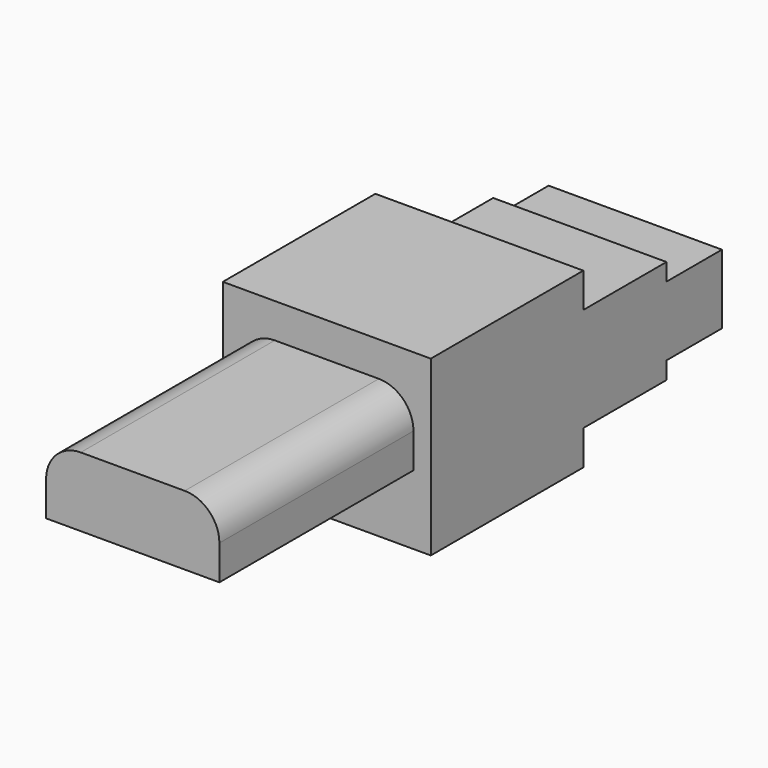
from build123d import *

# Parameters (mm, degrees)
F1_DEPTH = 7
F2_W     = 6
F2_H     = 5
F3_DEPTH = 5.5
F4_W     = 6
F4_H     = 3
F5_DEPTH = 3
F6_W     = 6
F6_H     = 2
F7_DEPTH = 2
F9_DEPTH = 1
F10_SIZE = 0.99999


# Not quite as in the source:
# - a fillet or chamfer is up to 0.001 mm smaller than in the source, because OpenCascade refuses the exact size


with BuildPart() as f1:
    # F0 (on Front) → F1 (new body)
    with BuildSketch(Plane.XZ):
        with BuildLine():
            Line((-2.5, -1), (2.5, -1))
            Line((2.5, -1), (2.5, 0))
            ThreePointArc((2.5, 0), (2.2071067812, 0.7071067812), (1.5, 1))
            Line((1.5, 1), (-1.5, 1))
            ThreePointArc((-1.5, 1), (-2.2071067812, 0.7071067812), (-2.5, 0))
            Line((-2.5, 0), (-2.5, -1))
        make_face()
    extrude(amount=F1_DEPTH)

    # F2 (on face) → F3 (join)
    with BuildSketch(Plane(origin=(0, 0, 0), x_dir=(-1, 0, 0), z_dir=(0, 1, 0))):
        with Locations((0, -0.5)):
            Rectangle(F2_W, F2_H)
        with BuildLine():
            ThreePointArc((1.5, 1), (2.2071067812, 0.7071067812), (2.5, 0))
            Line((2.5, 0), (2.5, -1))
            Line((2.5, -1), (-2.5, -1))
            Line((-2.5, -1), (-2.5, 0))
            ThreePointArc((-2.5, 0), (-2.2071067812, 0.7071067812), (-1.5, 1))
            Line((-1.5, 1), (1.5, 1))
        make_face(mode=Mode.SUBTRACT)
        with BuildLine():
            Line((2.5, -1), (2.5, 0))
            ThreePointArc((2.5, 0), (2.2071067812, 0.7071067812), (1.5, 1))
            Line((1.5, 1), (-1.5, 1))
            ThreePointArc((-1.5, 1), (-2.2071067812, 0.7071067812), (-2.5, 0))
            Line((-2.5, 0), (-2.5, -1))
            Line((-2.5, -1), (2.5, -1))
        make_face()
    extrude(amount=F3_DEPTH)

    # F4 (on face) → F5 (join)
    with BuildSketch(Plane(origin=(0, 5.5, 0), x_dir=(-1, 0, 0), z_dir=(0, 1, 0))):
        with Locations((0, -0.5)):
            Rectangle(F4_W, F4_H)
    extrude(amount=F5_DEPTH)

    # F6 (on face) → F7 (join)
    with BuildSketch(Plane(origin=(0, 8.5, 0), x_dir=(-1, 0, 0), z_dir=(0, 1, 0))):
        with Locations((0, -0.5)):
            Rectangle(F6_W, F6_H)
    extrude(amount=F7_DEPTH)

    # F8 (on face) → F9 (cut)
    with BuildSketch(Plane(origin=(-3, 0, 0), x_dir=(0, -1, 0), z_dir=(-1, 0, 0))):
        Polygon((-5.5, -2), (-5.5, 1), (-8.5, 1), (-8.5, 0.5), (-10.5, 0.5), (-10.5, -1.5), (-8.5, -1.5), (-8.5, -2), align=None)
    extrude(amount=-F9_DEPTH, mode=Mode.SUBTRACT)

    # F10 (size 1 in the source; OpenCascade refuses exactly that, so slightly less here)
    f10_edges = [f1.edges().sort_by_distance(p)[0] for p in [
        (-2, 5.5, -0.5),
    ]]
    chamfer(f10_edges, length=F10_SIZE)


solid = f1.part
